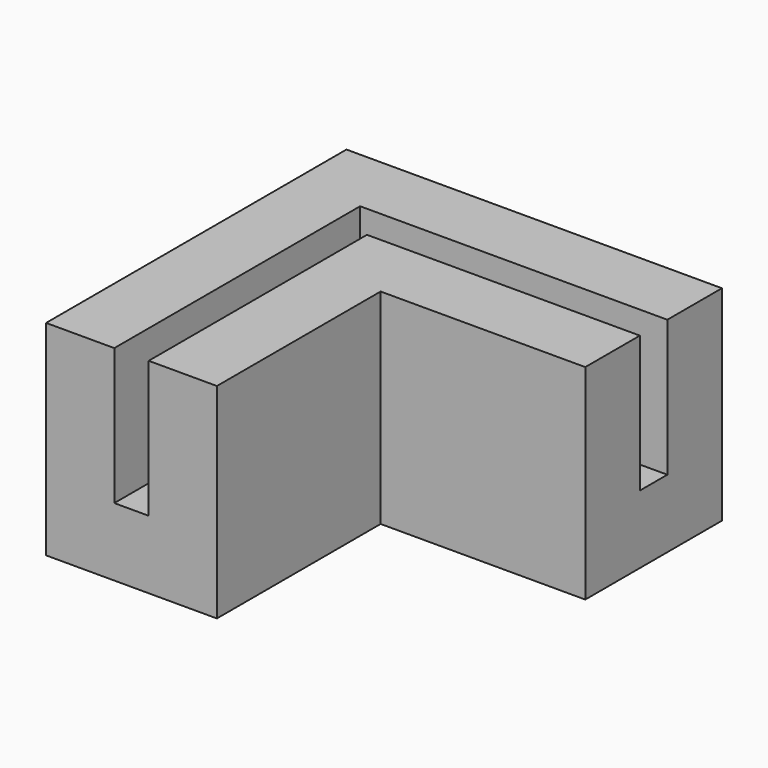
from build123d import *

# Parameters (mm, degrees)
F1_DEPTH = 6.35
F2_DEPTH = 12.7


# Not quite as in the source:
# - a feature names something its author has since deleted; it is built from what else it names


with BuildPart() as f1:
    # F0 (on Top) → F1 (new body)
    with BuildSketch(Plane.XY):
        Polygon((1.6, 1.6), (27, 1.6), (27, 7.95), (7.95, 7.95), (-7.95, 7.95), (-7.95, -7.95), (-7.95, -27), (-1.6, -27), (-1.6, -1.6), (-1.6, 1.6), align=None)
        Polygon((27, -7.95), (27, -1.6), (1.6, -1.6), (1.6, -27), (7.95, -27), (7.95, -7.95), align=None)
        Polygon((27, 0), (27, 1.6), (1.6, 1.6), (-1.6, 1.6), (-1.6, -1.6), (-1.6, -27), (0, -27), (1.6, -27), (1.6, -1.6), (27, -1.6), align=None)
    extrude(amount=-F1_DEPTH)

    # F0 (on Top) → F2 (join)
    with BuildSketch(Plane.XY):
        Polygon((1.6, 1.6), (27, 1.6), (27, 7.95), (7.95, 7.95), (-7.95, 7.95), (-7.95, -7.95), (-7.95, -27), (-1.6, -27), (-1.6, -1.6), (-1.6, 1.6), align=None)
        Polygon((27, -7.95), (27, -1.6), (1.6, -1.6), (1.6, -27), (7.95, -27), (7.95, -7.95), align=None)
    extrude(amount=F2_DEPTH)


solid = f1.part
